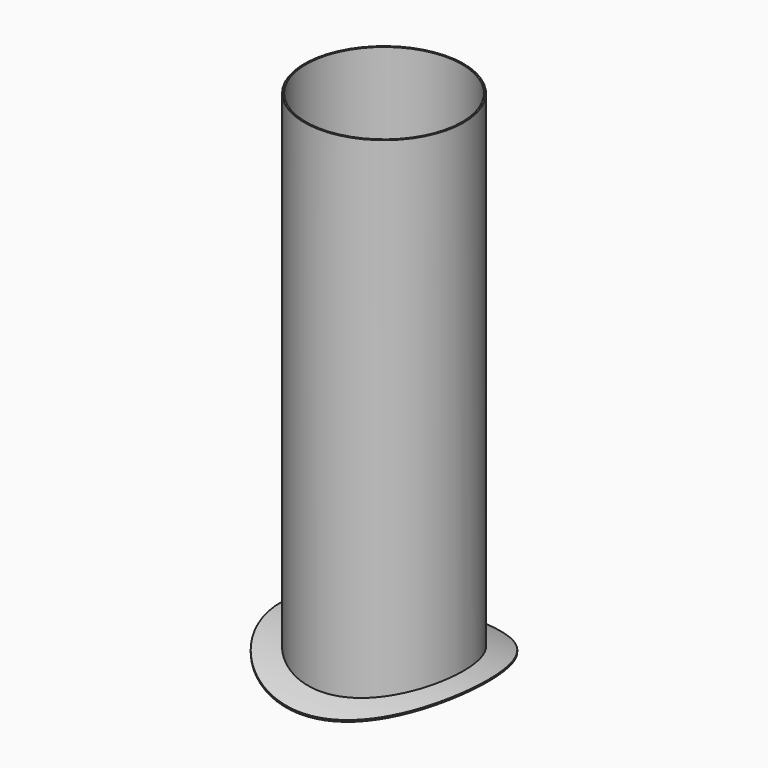
from build123d import *

# Parameters (mm, degrees)
F1_DEPTH      = 125
F1_DEPTH_BACK = 125
F2_R          = 250
F2_R_2        = 100
F2_R_3        = 75
F3_DEPTH      = 36.501
F5_R          = 76.5
F5_R_2        = 75
F6_REACH      = 700.9678513202


with BuildPart() as f1:
    # F0 (on Right) → F1 (new body, two sides)
    with BuildSketch(Plane.YZ) as f1_sk:
        with BuildLine():
            ThreePointArc((-131.6244658109, 0), (0, 35), (131.6244658109, 0))
            Line((131.6244658109, 0), (134.6189065473, 0))
            ThreePointArc((134.6189065473, 0), (0, 36.5), (-134.6189065473, 0))
            Line((-134.6189065473, 0), (-131.6244658109, 0))
        make_face()
    extrude(amount=F1_DEPTH)
    extrude(f1_sk.sketch, amount=-F1_DEPTH_BACK)

    # F2 (on Top) → F3 (cut, through all)
    with BuildSketch(Plane.XY):
        Circle(F2_R)
        Circle(F2_R_2, mode=Mode.SUBTRACT)
        Circle(F2_R_3)
    extrude(amount=F3_DEPTH, mode=Mode.SUBTRACT)

    f6_end = f1.faces().sort_by_distance((-97.1648773409, 0, 36.5))[0]
    # F5 (on offset) → F6 (join, up to a face of the model that its end follows)
    with BuildSketch(Plane.XY.offset(500)):
        Circle(F5_R)
        Circle(F5_R_2, mode=Mode.SUBTRACT)
    f6_long = extrude(amount=-F6_REACH, mode=Mode.PRIVATE)
    add(split(f6_long, bisect_by=f6_end, keep=Keep.TOP, mode=Mode.PRIVATE))


solid = f1.part
